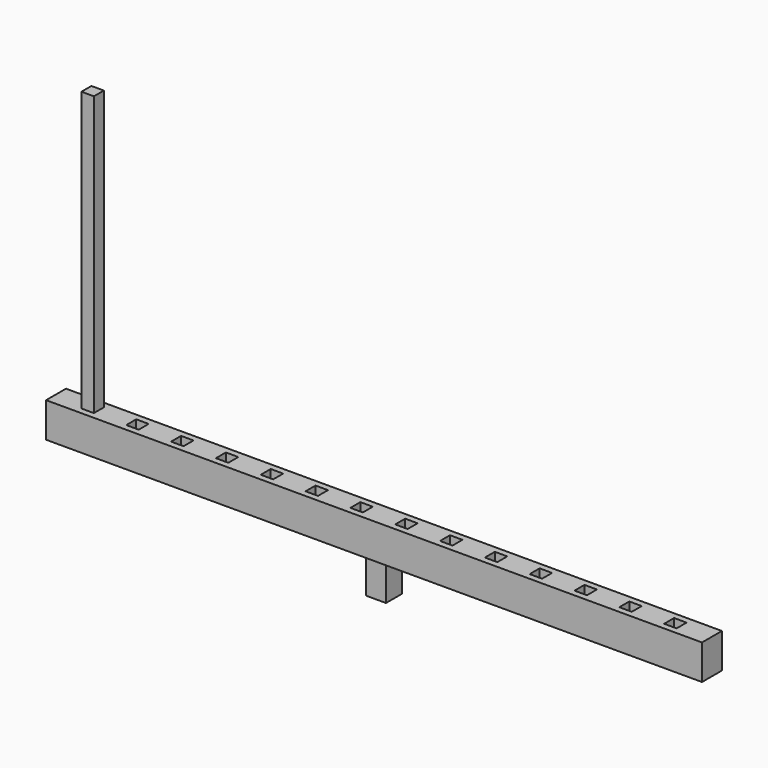
from build123d import *

# Parameters (mm, degrees)
F0_W     = 1672.59
F0_H     = 63.5
F0_W_2   = 31.75
F0_H_2   = 31.75
F1_DEPTH = 88.9
F3_W     = 50.8
F3_H     = 50.8
F4_DEPTH = 88.9
F2_W     = 31.75
F2_H     = 31.75
F5_DEPTH = 711.2


with BuildPart() as f1:
    # F0 (on Top) → F1 (new body)
    with BuildSketch(Plane.XY):
        Rectangle(F0_W, F0_H)
        with Locations((-742.95, 0)):
            Rectangle(F0_W_2, F0_H_2, mode=Mode.SUBTRACT)
        with Locations((-628.65, 0)):
            Rectangle(F0_W_2, F0_H_2, mode=Mode.SUBTRACT)
        with Locations((-514.35, 0)):
            Rectangle(F0_W_2, F0_H_2, mode=Mode.SUBTRACT)
        with Locations((-400.05, 0)):
            Rectangle(F0_W_2, F0_H_2, mode=Mode.SUBTRACT)
        with Locations((-285.75, 0)):
            Rectangle(F0_W_2, F0_H_2, mode=Mode.SUBTRACT)
        with Locations((-171.45, 0)):
            Rectangle(F0_W_2, F0_H_2, mode=Mode.SUBTRACT)
        with Locations((-57.15, 0)):
            Rectangle(F0_W_2, F0_H_2, mode=Mode.SUBTRACT)
        with Locations((57.15, 0)):
            Rectangle(F0_W_2, F0_H_2, mode=Mode.SUBTRACT)
        with Locations((171.45, 0)):
            Rectangle(F0_W_2, F0_H_2, mode=Mode.SUBTRACT)
        with Locations((285.75, 0)):
            Rectangle(F0_W_2, F0_H_2, mode=Mode.SUBTRACT)
        with Locations((400.05, 0)):
            Rectangle(F0_W_2, F0_H_2, mode=Mode.SUBTRACT)
        with Locations((514.35, 0)):
            Rectangle(F0_W_2, F0_H_2, mode=Mode.SUBTRACT)
        with Locations((628.65, 0)):
            Rectangle(F0_W_2, F0_H_2, mode=Mode.SUBTRACT)
        with Locations((742.95, 0)):
            Rectangle(F0_W_2, F0_H_2, mode=Mode.SUBTRACT)
    extrude(amount=F1_DEPTH)

    # F3 (on face) → F4 (join)
    with BuildSketch(Plane(origin=(0, 0, 0), x_dir=(1, 0, 0), z_dir=(0, 0, -1))):
        Rectangle(F3_W, F3_H)
    extrude(amount=F4_DEPTH)


with BuildPart() as f5:
    # F2 (on face) → F5 (new body)
    with BuildSketch(Plane.XY.offset(88.9)):
        with Locations((-742.95, 0)):
            Rectangle(F2_W, F2_H)
    extrude(amount=F5_DEPTH)


solid = Compound([f1.part, f5.part])
